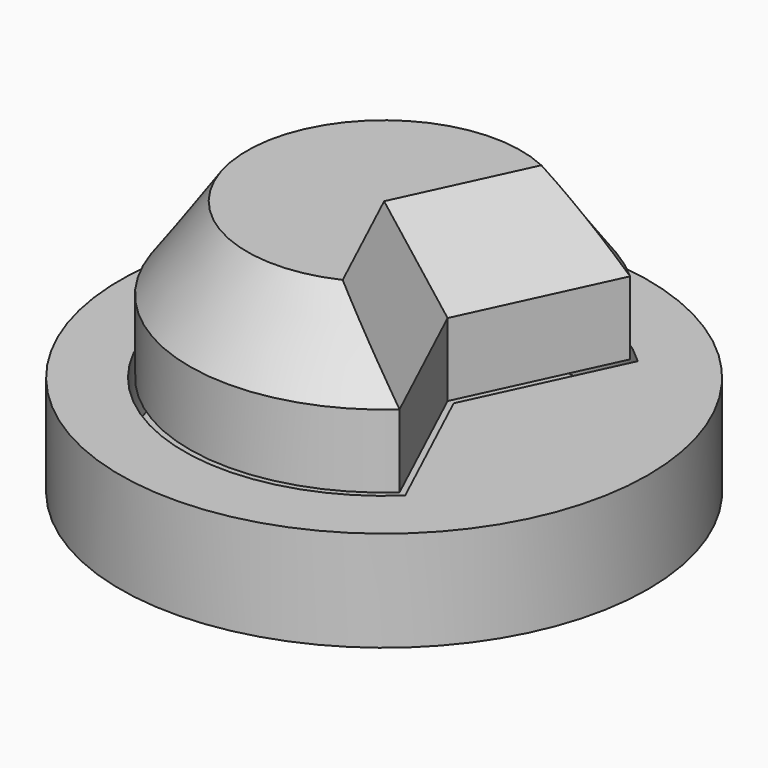
from build123d import *

# Parameters (mm, degrees)
F1_DEPTH               = 4.5
DRAFT_F1_DRAFTED_ANGLE = -35
F2_DEPTH               = 4
F3_R                   = 14.4509339219
F4_DEPTH               = 5.5
F5_DEPTH               = 3.75
F7_DEPTH               = 0.5
F8_DEPTH               = 3.75


# Not quite as in the source:
# - an extrude with a draft is written as a straight extrude whose walls are then drafted


with BuildPart() as f1:
    # F0 (on Top) → F1 (new body)
    with BuildSketch(Plane.XY):
        with BuildLine():
            Line((0, 0), (3.1696369631, 6.7973084028))
            ThreePointArc((3.1696369631, 6.7973084028), (-7.5, 0), (3.1696369631, -6.7973084028))
            Line((3.1696369631, -6.7973084028), (0, 0))
        make_face()
    extrude(amount=-F1_DEPTH)

    # draft_F1_drafted
    draft_f1_drafted_walls = [f1.faces().sort_by_distance(p)[0] for p in [
        (1.5848184815, -3.3986542014, -3),
        (1.5848184815, 3.3986542014, -3),
        (-7.5, 0, -3),
    ]]
    draft(draft_f1_drafted_walls, neutral_plane=Plane(origin=(0, 0, 0), x_dir=(1, 0, 0), z_dir=(0, 0, -1)), angle=DRAFT_F1_DRAFTED_ANGLE)

    # F2 (add): a face of the model
    f2_faces = [f1.faces().sort_by_distance(p)[0] for p in [
        (-1.7270371473, 0, -4.5),
    ]]
    extrude(f2_faces, amount=F2_DEPTH)

    # F3 (on face) → F8 (cut)
    with BuildSketch(Plane(origin=(0, 0, -8.5), x_dir=(1, 0, 0), z_dir=(0, 0, -1))):
        with BuildLine():
            Line((7.5198709308, -7.9608099429), (3.8076842893, 0))
            Line((3.8076842893, 0), (7.5198709308, 7.9608099429))
            ThreePointArc((7.5198709308, 7.9608099429), (-10.9509339219, 0), (7.5198709308, -7.9608099429))
        make_face()
        with BuildLine():
            Line((7.1555116732, 7.8892994685), (3.4766709136, 0))
            Line((3.4766709136, 0), (7.1555116732, -7.8892994685))
            ThreePointArc((7.1555116732, -7.8892994685), (-10.6509339219, 0), (7.1555116732, 7.8892994685))
        make_face(mode=Mode.SUBTRACT)
    extrude(amount=F8_DEPTH, mode=Mode.SUBTRACT)


with BuildPart() as f4:
    # F3 (on face) → F4 (new body)
    with BuildSketch(Plane(origin=(0, 0, -8.5), x_dir=(1, 0, 0), z_dir=(0, 0, -1))):
        Circle(F3_R)
        with BuildLine():
            Line((7.5198709308, 7.9608099429), (3.8076842893, 0))
            Line((3.8076842893, 0), (7.5198709308, -7.9608099429))
            ThreePointArc((7.5198709308, -7.9608099429), (-10.9509339219, 0), (7.5198709308, 7.9608099429))
        make_face(mode=Mode.SUBTRACT)
        with BuildLine():
            Line((7.5198709308, -7.9608099429), (3.8076842893, 0))
            Line((3.8076842893, 0), (7.5198709308, 7.9608099429))
            ThreePointArc((7.5198709308, 7.9608099429), (-10.9509339219, 0), (7.5198709308, -7.9608099429))
        make_face()
        with BuildLine():
            Line((7.1555116732, 7.8892994685), (3.4766709136, 0))
            Line((3.4766709136, 0), (7.1555116732, -7.8892994685))
            ThreePointArc((7.1555116732, -7.8892994685), (-10.6509339219, 0), (7.1555116732, 7.8892994685))
        make_face(mode=Mode.SUBTRACT)
        with BuildLine():
            Line((7.1555116732, -7.8892994685), (3.4766709136, 0))
            Line((3.4766709136, 0), (7.1555116732, 7.8892994685))
            ThreePointArc((7.1555116732, 7.8892994685), (-10.6509339219, 0), (7.1555116732, -7.8892994685))
        make_face()
    extrude(amount=F4_DEPTH)

    # F3 (on face) → F5 (cut)
    with BuildSketch(Plane(origin=(0, 0, -8.5), x_dir=(1, 0, 0), z_dir=(0, 0, -1))):
        with BuildLine():
            Line((7.5198709308, -7.9608099429), (3.8076842893, 0))
            Line((3.8076842893, 0), (7.5198709308, 7.9608099429))
            ThreePointArc((7.5198709308, 7.9608099429), (-10.9509339219, 0), (7.5198709308, -7.9608099429))
        make_face()
        with BuildLine():
            Line((7.1555116732, 7.8892994685), (3.4766709136, 0))
            Line((3.4766709136, 0), (7.1555116732, -7.8892994685))
            ThreePointArc((7.1555116732, -7.8892994685), (-10.6509339219, 0), (7.1555116732, 7.8892994685))
        make_face(mode=Mode.SUBTRACT)
        with BuildLine():
            Line((7.1555116732, -7.8892994685), (3.4766709136, 0))
            Line((3.4766709136, 0), (7.1555116732, 7.8892994685))
            ThreePointArc((7.1555116732, 7.8892994685), (-10.6509339219, 0), (7.1555116732, -7.8892994685))
        make_face()
    extrude(amount=F5_DEPTH, mode=Mode.SUBTRACT)

    # F6 (on face) → F7 (cut)
    with BuildSketch(Plane(origin=(0, 0, -14), x_dir=(1, 0, 0), z_dir=(0, 0, -1))):
        with BuildLine():
            Line((3.8076842893, 0), (7.5198709308, 7.9608099429))
            ThreePointArc((7.5198709308, 7.9608099429), (-10.9509339219, 0), (7.5198709308, -7.9608099429))
            Line((7.5198709308, -7.9608099429), (3.8076842893, 0))
        make_face()
    extrude(amount=-F7_DEPTH, mode=Mode.SUBTRACT)


solid = Compound([f1.part, f4.part])
